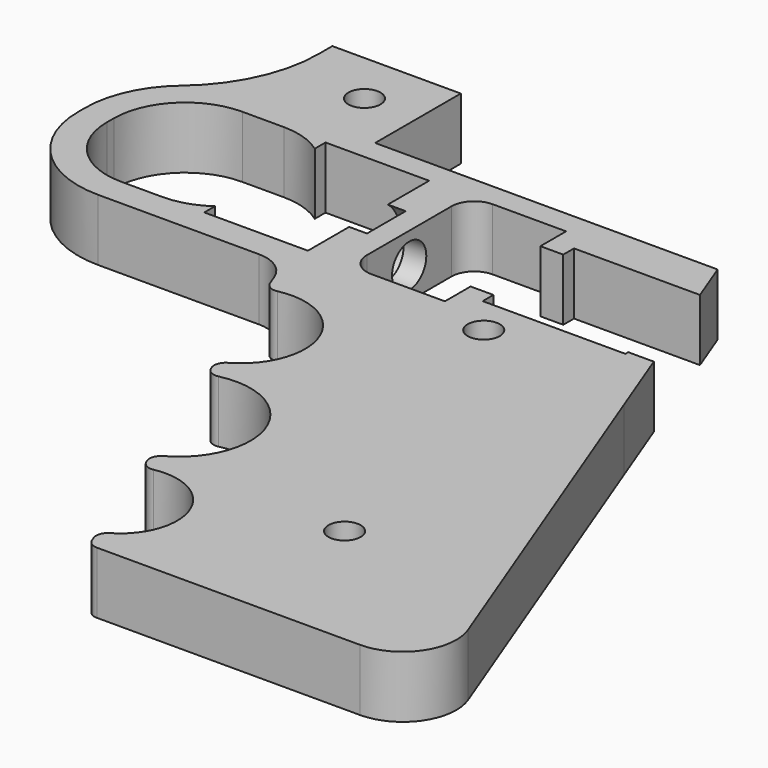
from build123d import *

# Parameters (mm, degrees)
F0_R     = 2.25
F1_DEPTH = 4.330125
F2_W     = 20
F2_H     = 16
F3_DEPTH = 12.5
F4_R     = 3.2
F5_W     = 6.4
F5_H     = 8.66025
F5_R     = 3
F6_DEPTH = 3.2
F8_DEPTH = 2.5
F9_R     = 1.6
F10_R    = 5


# Not quite as in the source:
# - ends of sketch curves that miss each other by under 0.0002 mm in the source are joined


with BuildPart() as f1:
    # F0 (on Top) → F1 (new body, symmetric)
    with BuildSketch(Plane.XY):
        with BuildLine():
            Line((20, -24.8214285714), (0, 27.4853587511))
            Line((0, 27.4853587511), (-3.829193786, 37.5))
            Line((-3.829193786, 37.5), (-12.6123318144, 37.5))
            Line((-12.6123318144, 37.5), (-25.6123318144, 37.5))
            Line((-25.6123318144, 37.5), (-25.6123318144, 38.8834841531))
            Line((-25.6123318144, 38.8834841531), (-30.6123318144, 38.8834841531))
            Line((-30.6123318144, 38.8834841531), (-30.6123318144, 34.3834841531))
            Line((-30.6123318144, 34.3834841531), (-44.1123318144, 34.3834841531))
            Line((-44.1123318144, 34.3834841531), (-44.1123318144, 41.8))
            Line((-44.1123318144, 41.8), (-47.3123318144, 41.8))
            Line((-47.3123318144, 41.8), (-47.3123318144, 34.3834841531))
            Line((-47.3123318144, 34.3834841531), (-64.3336698413, 34.3834841531))
            Line((-64.3336698413, 34.3834841531), (-64.3336698413, 36.2610286334))
            ThreePointArc((-64.3336698413, 36.2610286334), (-67.1028911134, 34.8644323695), (-70.1668349206, 34.3834792274))
            Line((-70.1668349206, 34.3834792274), (-76, 34.3834841531))
            ThreePointArc((-76, 34.3834841531), (-83.0710678119, 37.3124163412), (-86, 44.3834841531))
            Line((-86, 44.3834841531), (-86, 45.6165158469))
            ThreePointArc((-86, 45.6165158469), (-83.0710678119, 52.6875836588), (-76, 55.6165158469))
            Line((-76, 55.6165158469), (-70.1668349206, 55.6165158469))
            ThreePointArc((-70.1668349206, 55.6165158469), (-67.1028911134, 55.1355676305), (-64.3336698413, 53.7389713666))
            Line((-64.3336698413, 53.7389713666), (-64.3336698413, 55.6165158469))
            Line((-64.3336698413, 55.6165158469), (-47.3123318144, 55.6165158469))
            Line((-47.3123318144, 55.6165158469), (-47.3123318144, 48.2))
            Line((-47.3123318144, 48.2), (-44.1123318144, 48.2))
            Line((-44.1123318144, 48.2), (-44.1123318144, 55.6165158469))
            Line((-44.1123318144, 55.6165158469), (-30.6123318144, 55.6165158469))
            Line((-30.6123318144, 55.6165158469), (-30.6123318144, 51.1165158469))
            Line((-30.6123318144, 51.1165158469), (-25.6123318144, 51.1165158469))
            Line((-25.6123318144, 51.1165158469), (-25.6123318144, 52.5))
            Line((-25.6123318144, 52.5), (-12.6123318144, 52.5))
            Line((-12.6123318144, 52.5), (-9.5645871327, 52.5))
            Line((-9.5645871327, 52.5), (-12.0202176002, 58.9223070303))
            Line((-12.0202176002, 58.9223070303), (-60.0202176002, 58.9223070303))
            Line((-60.0202176002, 58.9223070303), (-60.0202176002, 73.9223070303))
            Line((-60.0202176002, 73.9223070303), (-78.0202176002, 73.9223070303))
            Line((-78.0202176002, 73.9223070303), (-78.0202176002, 71.5223070303))
            ThreePointArc((-78.0202176002, 71.5223070303), (-79.8672373555, 63.1277070855), (-85.0671484236, 56.2836063342))
            ThreePointArc((-85.0671484236, 56.2836063342), (-88.7070861713, 51.4927358083), (-90, 45.6165158469))
            Line((-90, 45.6165158469), (-90, 44.3834841531))
            ThreePointArc((-90, 44.3834841531), (-85.8994949366, 34.4839892165), (-76, 30.3834841531))
            Line((-76, 30.3834841531), (-50, 30.3834841531))
            Line((-50, 30.3834841531), (-47.7142857143, 24.405565602))
            ThreePointArc((-47.7142857143, 24.405565602), (-36.0935520375, 19.2134033537), (-41.2857142857, 7.5926696769))
            Line((-41.2857142857, 7.5926696769), (-40.1428571429, 4.6037104013))
            ThreePointArc((-40.1428571429, 4.6037104013), (-27.2309308353, -1.1653587634), (-33, -14.077285071))
            Line((-33, -14.077285071), (-31.8571428571, -17.0662443466))
            ThreePointArc((-31.8571428571, -17.0662443466), (-21.5276018111, -21.6814996784), (-26.1428571429, -32.0110407244))
            Line((-26.1428571429, -32.0110407244), (-25, -35))
            Line((-25, -35), (12.9946266979, -35))
            ThreePointArc((12.9946266979, -35), (19.1727852307, -31.7521003214), (20, -24.8214285714))
        make_face()
        with Locations((-5.1674522335, -15)):
            Circle(F0_R, mode=Mode.SUBTRACT)
        with Locations((-67.5202176002, 66.4223070303)):
            Circle(F0_R, mode=Mode.SUBTRACT)
        with Locations((-23.0245950907, 31.7024886808)):
            Circle(F0_R, mode=Mode.SUBTRACT)
    extrude(amount=F1_DEPTH, both=True)

    # F2 (on Top) → F3 (cut, symmetric)
    with BuildSketch(Plane.XY):
        with Locations((-17.4123318144, 45)):
            Rectangle(F2_W, F2_H)
    extrude(amount=F3_DEPTH, both=True, mode=Mode.SUBTRACT)

    # F4
    f4_edges = [f1.edges().sort_by_distance(p)[0] for p in [
        (-44.112332, 55.616516, 0),
        (-44.112332, 34.383484, 0),
    ]]
    fillet(f4_edges, radius=F4_R)

    # F5 (on face) → F6 (join)
    with BuildSketch(Plane.YZ.offset(-44.1123318144)):
        with Locations((45, 0)):
            Rectangle(F5_W, F5_H)
        with Locations((45, 0)):
            Circle(F5_R, mode=Mode.SUBTRACT)
    extrude(amount=-F6_DEPTH)

    # F7 (on face) → F8 (join)
    with BuildSketch(Plane(origin=(-47.3123318144, 0, 0), x_dir=(0, -1, 0), z_dir=(-1, 0, 0))):
        with BuildLine():
            Line((-48.3911675695, 4.330125), (-55.6165158469, 4.330125))
            Line((-55.6165158469, 4.330125), (-55.6165158469, -4.330125))
            Line((-55.6165158469, -4.330125), (-48.3911675695, -4.330125))
            ThreePointArc((-48.3911675695, -4.330125), (-50.5, 0), (-48.3911675695, 4.330125))
        make_face()
        with BuildLine():
            Line((-34.3834841531, -4.330125), (-34.3834841531, 4.330125))
            Line((-34.3834841531, 4.330125), (-41.6088324305, 4.330125))
            ThreePointArc((-41.6088324305, 4.330125), (-39.5, 0), (-41.6088324305, -4.330125))
            Line((-41.6088324305, -4.330125), (-34.3834841531, -4.330125))
        make_face()
    extrude(amount=F8_DEPTH)

    # F9
    f9_edges = [f1.edges().sort_by_distance(p)[0] for p in [
        (-25, -35, 0),
        (-26.142857, -32.011041, 0),
        (-31.857143, -17.066244, 0),
        (-33, -14.077285, 0),
        (-40.142857, 4.60371, 0),
        (-41.285714, 7.59267, 0),
        (-47.714286, 24.405566, 0),
    ]]
    fillet(f9_edges, radius=F9_R)

    # F10
    f10_edges = [f1.edges().sort_by_distance(p)[0] for p in [
        (-50, 30.383484, 0),
    ]]
    fillet(f10_edges, radius=F10_R)


solid = f1.part
